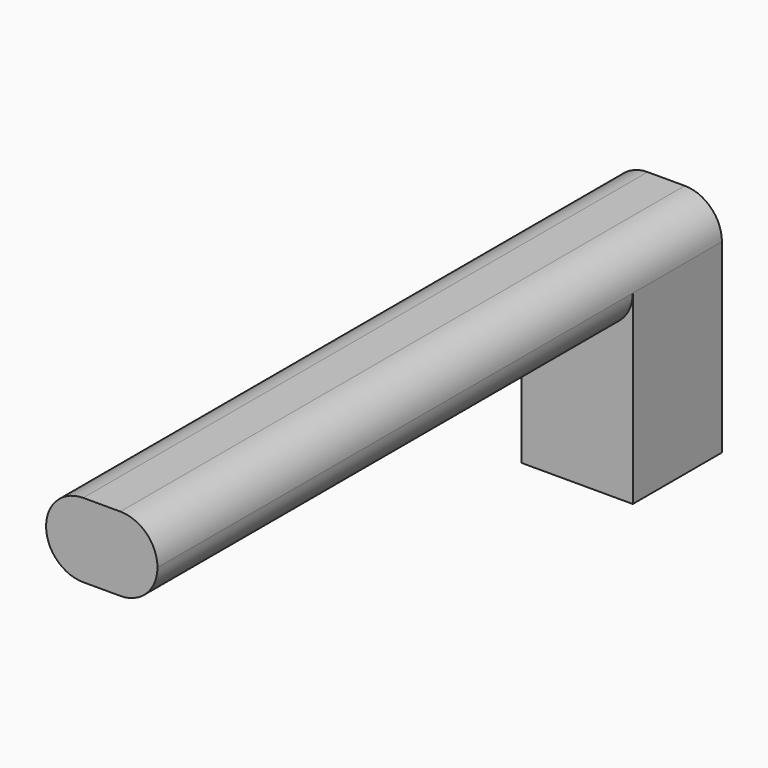
from build123d import *

# Parameters (mm, degrees)
F0_W     = 15
F0_H     = 15
F1_DEPTH = 30
F2_W     = 15
F2_H     = 10
F3_DEPTH = 80
F4_R     = 4.99999
F5_W     = 10
F5_H     = 10
F6_DEPTH = 20


# Not quite as in the source:
# - a fillet or chamfer is up to 0.001 mm smaller than in the source, because OpenCascade refuses the exact size


with BuildPart() as f1:
    # F0 (on Top) → F1 (new body)
    with BuildSketch(Plane.XY):
        Rectangle(F0_W, F0_H)
    extrude(amount=F1_DEPTH)

    # F2 (on face) → F3 (join)
    with BuildSketch(Plane.XZ.offset(7.5)):
        with Locations((0, 25)):
            Rectangle(F2_W, F2_H)
    extrude(amount=F3_DEPTH)

    # F4 (radius 5 in the source; OpenCascade refuses exactly that, so slightly less here)
    f4_edges = [f1.edges().sort_by_distance(p)[0] for p in [
        (7.5, -40, 30),
        (-7.5, -40, 30),
        (7.5, -47.5, 20),
        (-7.5, -47.5, 20),
    ]]
    fillet(f4_edges, radius=F4_R)

    # F5 (on face) → F6 (cut)
    with BuildSketch(Plane(origin=(0, 0, 0), x_dir=(1, 0, 0), z_dir=(0, 0, -1))):
        Rectangle(F5_W, F5_H)
    extrude(amount=-F6_DEPTH, mode=Mode.SUBTRACT)


solid = f1.part
